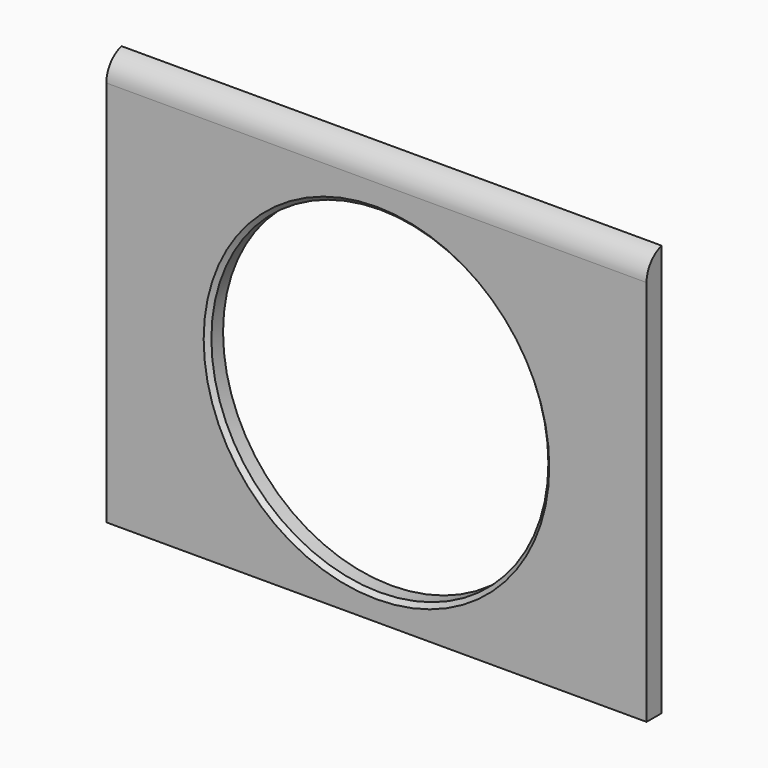
from build123d import *

# Parameters (mm, degrees)
F0_W        = 630
F0_H        = 480
F0_R        = 196.5
F1_DEPTH    = 22
F2_T1_DEPTH = 774.568322948
F3_SIZE     = 5


# Not quite as in the source:
# - a fillet or chamfer that OpenCascade refuses, or shapes differently, is made with other operations: its cross-section is extruded or revolved along the edge and cut away or added


with BuildPart() as f1:
    # F0 (on Front) → F1 (new body)
    with BuildSketch(Plane.XZ):
        Rectangle(F0_W, F0_H)
        with Locations((0, -15)):
            Circle(F0_R, mode=Mode.SUBTRACT)
    extrude(amount=F1_DEPTH)

    # F2: fillet of radius 30 on 1 edges, made by hand

    # F2_s2 → F2_t1 (cut)
    with BuildSketch(Plane.YZ.offset(-387.284161474)):
        with BuildLine():
            ThreePointArc((0, 240), (-15.8746727726, 229.252237535), (-22, 211.0863354104))
            Line((-22, 211.0863354104), (-22, 240))
            Line((-22, 240), (0, 240))
        make_face()
    extrude(amount=F2_T1_DEPTH, mode=Mode.SUBTRACT)

    # F3
    f3_edges = [f1.edges().sort_by_distance(p)[0] for p in [
        (-196.5, -22, -15),
    ]]
    chamfer(f3_edges, length=F3_SIZE)


solid = f1.part
